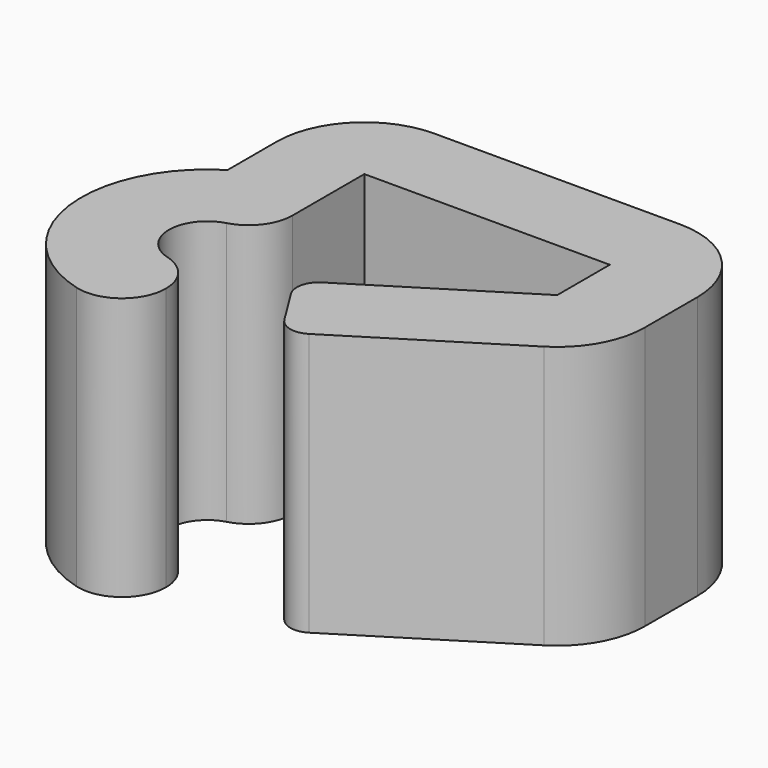
from build123d import *

# Parameters (mm, degrees)
F1_DEPTH = 6
F2_R     = 0.99999


# Not quite as in the source:
# - a fillet or chamfer is up to 0.001 mm smaller than in the source, because OpenCascade refuses the exact size


with BuildPart() as f1:
    # F0 (on Top) → F1 (new body)
    with BuildSketch(Plane.XY):
        with BuildLine():
            Line((-79.3681601882, 18.7270958871), (-79.3681601882, 21.703983524))
            Line((-79.3681601882, 21.703983524), (-73.7681601882, 21.703983524))
            Line((-73.7681601882, 21.703983524), (-73.7681601882, 20.203983524))
            Line((-73.7681601882, 20.203983524), (-77.3441610362, 17.968982994))
            ThreePointArc((-77.3441610362, 17.968982994), (-77.566357164, 17.6574135954), (-77.5031607182, 17.279984372))
            Line((-77.5031607182, 17.279984372), (-76.9731617782, 16.431986068))
            ThreePointArc((-76.9731617782, 16.431986068), (-76.6615923795, 16.2097899402), (-76.2841631562, 16.272986386))
            Line((-76.2841631562, 16.272986386), (-72.7081623082, 18.507986916))
            ThreePointArc((-72.7081623082, 18.507986916), (-72.0188752257, 19.2344464592), (-71.7681601882, 20.203983524))
            Line((-71.7681601882, 20.203983524), (-71.7681601882, 21.703983524))
            ThreePointArc((-71.7681601882, 21.703983524), (-72.3539466258, 23.1181970864), (-73.7681601882, 23.703983524))
            Line((-73.7681601882, 23.703983524), (-79.3681601882, 23.703983524))
            ThreePointArc((-79.3681601882, 23.703983524), (-80.7823737506, 23.1181970864), (-81.3681601882, 21.703983524))
            Line((-81.3681601882, 21.703983524), (-81.3681601882, 20.3047729959))
            ThreePointArc((-81.3681601882, 20.3047729959), (-82.5569903042, 16.8343446369), (-79.3681601882, 15.0209079738))
            Line((-79.3681601882, 15.0209079738), (-79.3681601882, 16.9770958871))
            Line((-79.3681601882, 16.9770958871), (-79.8681601882, 16.9770958871))
            ThreePointArc((-79.8681601882, 16.9770958871), (-80.7431601882, 17.8520958871), (-79.8681601882, 18.7270958871))
            Line((-79.8681601882, 18.7270958871), (-79.3681601882, 18.7270958871))
        make_face()
    extrude(amount=F1_DEPTH)

    # F2 (radius 1 in the source; OpenCascade refuses exactly that, so slightly less here)
    f2_edges = [f1.edges().sort_by_distance(p)[0] for p in [
        (-79.36816, 15.020908, 3),
        (-79.36816, 18.727096, 3),
        (-79.36816, 16.977096, 3),
    ]]
    fillet(f2_edges, radius=F2_R)


solid = f1.part
